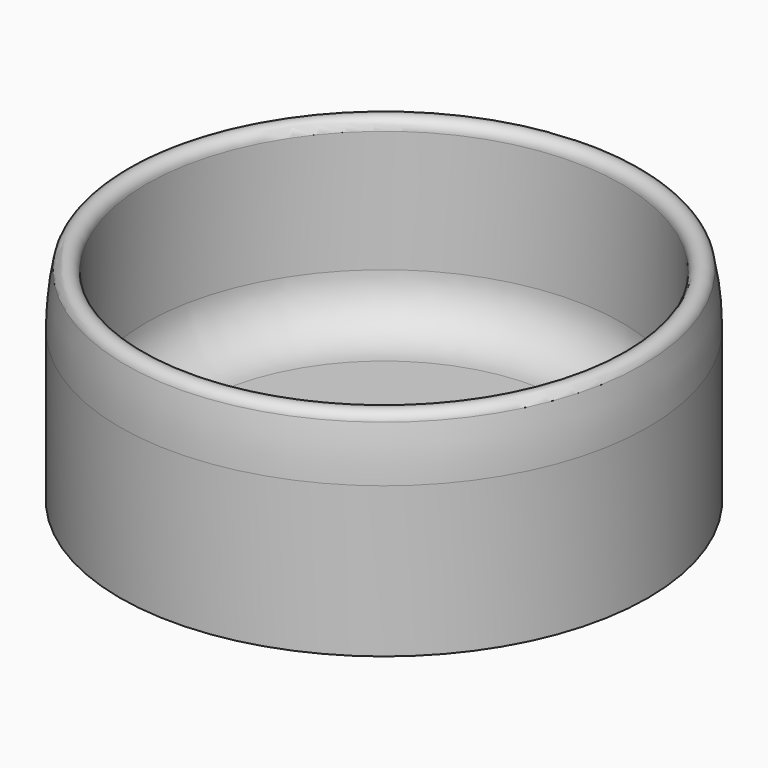
from build123d import *

# Parameters (mm, degrees)
F0_R     = 50
F1_DEPTH = 50
F2_T     = -5
F5_R     = 10


# Not quite as in the source:
# - a fillet or chamfer that OpenCascade refuses, or shapes differently, is made with other operations: its cross-section is extruded or revolved along the edge and cut away or added


with BuildPart() as f1:
    # F0 (on Top) → F1 (new body)
    with BuildSketch(Plane.XY):
        with Locations((-0.0575962756, 0.3432892042)):
            Circle(F0_R)
    extrude(amount=F1_DEPTH)

    # F2
    f2_openings = [f1.faces().sort_by_distance(p)[0] for p in [
        (-0.057596, 0.343289, 50),
    ]]
    offset(amount=F2_T, openings=f2_openings)

    # F3: fillet of radius 49 on 1 edges, made by hand

    # F3_s1 → F3_t2 (revolve, cut)
    with BuildSketch(Plane.XZ.offset(-0.3432892042)):
        with BuildLine():
            ThreePointArc((49.9424037244, 28.4361413472), (48.6760396639, 39.5041131577), (44.9424037244, 50))
            Line((44.9424037244, 50), (49.9424037244, 50))
            Line((49.9424037244, 50), (49.9424037244, 28.4361413472))
        make_face()
    revolve(axis=Axis((-0.0575962756, 0.3432892042, 50), (0, 0, 1)), mode=Mode.SUBTRACT)

    # F4: fillet of radius 2 on 1 edges, made by hand

    # F4_s1 → F4_t2 (revolve, cut)
    with BuildSketch(Plane.XZ.offset(-0.3432892042)):
        with BuildLine():
            ThreePointArc((48.8998505329, 38.4901602258), (46.7361194752, 40.0691253656), (44.9424037244, 38.0797921083))
            Line((44.9424037244, 38.0797921083), (44.9424037244, 50))
            ThreePointArc((44.9424037244, 50), (47.2798843291, 44.3684321809), (48.8998505329, 38.4901602258))
        make_face()
    revolve(axis=Axis((-0.0575962756, 0.3432892042, 50), (0, 0, 1)), mode=Mode.SUBTRACT)

    # F5
    f5_edges = [f1.edges().sort_by_distance(p)[0] for p in [
        (-45.057596, 0.343289, 5),
    ]]
    fillet(f5_edges, radius=F5_R)


solid = f1.part
